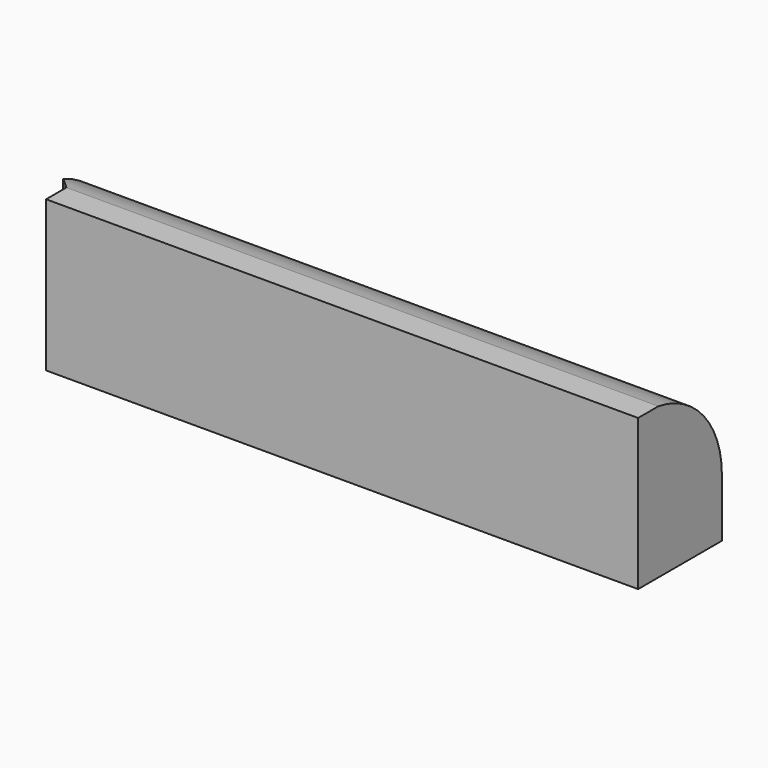
from build123d import *

# Parameters (mm, degrees)
F0_W        = 194.6241557598
F0_H        = 48.2458211482
F1_DEPTH    = 25.4
F2_T1_DEPTH = 343.5218255279
F3_SIZE     = 5.08
F4_W        = 189.5441557598
F4_H        = 48.2458211482
F5_DEPTH    = 8.1318449229


# Not quite as in the source:
# - a fillet or chamfer that OpenCascade refuses, or shapes differently, is made with other operations: its cross-section is extruded or revolved along the edge and cut away or added


with BuildPart() as f1:
    # F0 (on Front) → F1 (new body)
    with BuildSketch(Plane.XZ):
        with Locations((-97.3120778799, 84.4252165407)):
            Rectangle(F0_W, F0_H)
    extrude(amount=F1_DEPTH)

    # F2: fillet of radius 30.1570992617 on 1 edges, made by hand

    # F2_s2 → F2_t1 (cut)
    with BuildSketch(Plane.YZ.offset(-269.0729906439)):
        with BuildLine():
            ThreePointArc((-25.4, 108.5481271148), (-7.2124816956, 98.3388553113), (0, 78.7685931612))
            Line((0, 78.7685931612), (0, 108.5481271148))
            Line((0, 108.5481271148), (-25.4, 108.5481271148))
        make_face()
    extrude(amount=F2_T1_DEPTH, mode=Mode.SUBTRACT)

    # F3
    f3_edges = [f1.edges().sort_by_distance(p)[0] for p in [
        (-194.624156, -25.4, 84.425217),
    ]]
    chamfer(f3_edges, length=F3_SIZE)

    # F4 (on face) → F5 (join)
    with BuildSketch(Plane.XZ.offset(25.4)):
        with Locations((-94.7720778799, 84.4252165407)):
            Rectangle(F4_W, F4_H)
    extrude(amount=F5_DEPTH)


solid = f1.part
